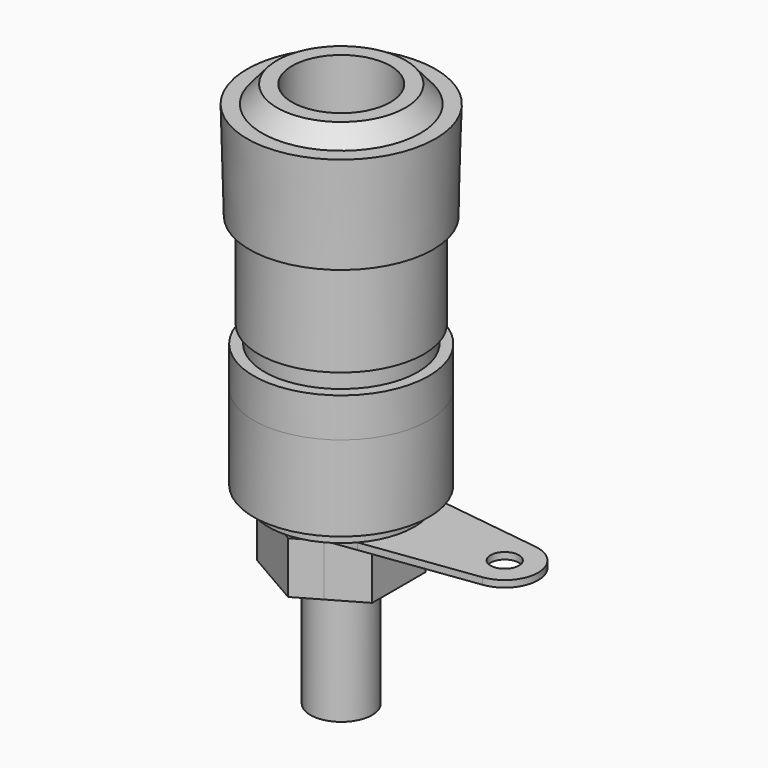
from build123d import *

# Parameters (mm, degrees)
F0_R      = 5.25
F0_R_2    = 3.925
F0_R_3    = 2.4
F1_DEPTH  = 2.35
F2_DEPTH  = 5
F3_DEPTH  = 5.1
F4_R      = 4.6
F4_R_2    = 2.85
F4_R_3    = 2.4
F4_R_4    = 2.35
F4_R_5    = 2
F5_DEPTH  = 1.05
F6_DEPTH  = 9.25
F4_R_6    = 1.85
F7_DEPTH  = 2.5
F8_DEPTH  = 19
F9_DEPTH  = 2.15
F12_R     = 4.375
F12_R_2   = 3.925
F12_R_3   = 2.1
F13_DEPTH = 0.8
F14_R     = 2.1
F14_R_2   = 0.85
F15_DEPTH = 0.4
F16_R     = 2.1
F16_R_2   = 1.7
F17_DEPTH = 3.1


with BuildPart() as f1:
    # F0 (on Top) → F1 (new body)
    with BuildSketch(Plane.XY):
        Circle(F0_R)
        Circle(F0_R_2, mode=Mode.SUBTRACT)
        Circle(F0_R_2)
        Circle(F0_R_3, mode=Mode.SUBTRACT)
    extrude(amount=F1_DEPTH)

    # F0 (on Top) → F2 (join)
    with BuildSketch(Plane.XY):
        Circle(F0_R_2)
        Circle(F0_R_3, mode=Mode.SUBTRACT)
    extrude(amount=-F2_DEPTH)


with BuildPart() as f3:
    # F0 (on Top) → F3 (new body)
    with BuildSketch(Plane.XY):
        Circle(F0_R)
        Circle(F0_R_2, mode=Mode.SUBTRACT)
    extrude(amount=-F3_DEPTH)


with BuildPart() as f5:
    # F4 (on face) → F5 (new body)
    with BuildSketch(Plane.XY.offset(2.35)):
        Circle(F4_R)
        Circle(F4_R_2, mode=Mode.SUBTRACT)
        Circle(F4_R_2)
        Circle(F4_R_3, mode=Mode.SUBTRACT)
        Circle(F4_R_3)
        Circle(F4_R_4, mode=Mode.SUBTRACT)
        Circle(F4_R_4)
        Circle(F4_R_5, mode=Mode.SUBTRACT)
    extrude(amount=F5_DEPTH)

    # F4 (on face) → F6 (join)
    with BuildSketch(Plane.XY.offset(2.35)):
        Circle(F4_R_2)
        Circle(F4_R_3, mode=Mode.SUBTRACT)
        Circle(F4_R_3)
        Circle(F4_R_4, mode=Mode.SUBTRACT)
        Circle(F4_R_4)
        Circle(F4_R_5, mode=Mode.SUBTRACT)
    extrude(amount=F6_DEPTH)

    # F4 (on face) → F7 (join)
    with BuildSketch(Plane.XY.offset(2.35)):
        Circle(F4_R_4)
        Circle(F4_R_5, mode=Mode.SUBTRACT)
        Circle(F4_R_5)
        Circle(F4_R_6, mode=Mode.SUBTRACT)
    extrude(amount=-F7_DEPTH)

    # F4 (on face) → F8 (join)
    with BuildSketch(Plane.XY.offset(2.35)):
        Circle(F4_R_6)
    extrude(amount=-F8_DEPTH)

    # F4 (on face) → F9 (cut)
    with BuildSketch(Plane.XY.offset(2.35)):
        Circle(F4_R_5)
        Circle(F4_R_6, mode=Mode.SUBTRACT)
        Circle(F4_R_6)
    extrude(amount=-F9_DEPTH, mode=Mode.SUBTRACT)


with BuildPart() as f11:
    # F10 (on Front) → F11 (revolve)
    with BuildSketch(Plane.XZ):
        Polygon((3.85, 16.05), (2.95, 16.05), (2.95, 11.55), (2.7, 11.55), (2.7, 6.8), (3.2, 6.8), (3.2, 3.4), (4.95, 3.4), (4.95, 9.1), (5.5, 9.1), (5.65, 15), (4.75, 15), align=None)
    revolve(axis=Axis((0, 0, 12.6171559095), (0, 0, 1)))


with BuildPart() as f13:
    # F12 (on face) → F13 (new body)
    with BuildSketch(Plane(origin=(0, 0, -5.1), x_dir=(1, 0, 0), z_dir=(0, 0, -1))):
        Circle(F12_R)
        Circle(F12_R_2, mode=Mode.SUBTRACT)
        Circle(F12_R_2)
        Circle(F12_R_3, mode=Mode.SUBTRACT)
    extrude(amount=F13_DEPTH)


with BuildPart() as f15:
    # F14 (on face) → F15 (new body)
    with BuildSketch(Plane(origin=(0, 0, -5.9), x_dir=(1, 0, 0), z_dir=(0, 0, -1))):
        with BuildLine():
            Line((0.437755102, -3.2708363564), (3.2847605668, -2.889805014))
            ThreePointArc((3.2847605668, -2.889805014), (4.0933758977, -1.5443117432), (4.375, 0))
            ThreePointArc((4.375, 0), (4.0933758977, 1.5443117432), (3.2847605668, 2.889805014))
            Line((3.2847605668, 2.889805014), (0.437755102, 3.2708363564))
            ThreePointArc((0.437755102, 3.2708363564), (-3.3, 0), (0.437755102, -3.2708363564))
        make_face()
        Circle(F14_R, mode=Mode.SUBTRACT)
        with BuildLine():
            Line((3.2847605668, -2.889805014), (10.0653061224, -1.9823250645))
            ThreePointArc((10.0653061224, -1.9823250645), (11.8, 0), (10.0653061224, 1.9823250645))
            Line((10.0653061224, 1.9823250645), (3.2847605668, 2.889805014))
            ThreePointArc((3.2847605668, 2.889805014), (4.0933758977, 1.5443117432), (4.375, 0))
            ThreePointArc((4.375, 0), (4.0933758977, -1.5443117432), (3.2847605668, -2.889805014))
        make_face()
        with Locations((9.8, 0)):
            Circle(F14_R_2, mode=Mode.SUBTRACT)
    extrude(amount=F15_DEPTH)


with BuildPart() as f17:
    # F16 (on face) → F17 (new body)
    with BuildSketch(Plane(origin=(0, 0, -6.3), x_dir=(1, 0, 0), z_dir=(0, 0, -1))):
        with BuildLine():
            Line((3.45, 1.9918584287), (1.4752466365, 3.1319828147))
            Line((1.4752466365, 3.1319828147), (0.437755102, 3.2708363564))
            ThreePointArc((0.437755102, 3.2708363564), (-3.3, 0), (0.437755102, -3.2708363564))
            Line((0.437755102, -3.2708363564), (1.4752466365, -3.1319828147))
            Line((1.4752466365, -3.1319828147), (3.45, -1.9918584287))
            Line((3.45, -1.9918584287), (3.45, 1.9918584287))
        make_face()
        Circle(F16_R, mode=Mode.SUBTRACT)
        Circle(F16_R)
        Circle(F16_R_2, mode=Mode.SUBTRACT)
        with BuildLine():
            Line((1.4752466365, 3.1319828147), (0, 3.9837168574))
            Line((0, 3.9837168574), (-3.45, 1.9918584287))
            Line((-3.45, 1.9918584287), (-3.45, -1.9918584287))
            Line((-3.45, -1.9918584287), (0, -3.9837168574))
            Line((0, -3.9837168574), (1.4752466365, -3.1319828147))
            Line((1.4752466365, -3.1319828147), (0.437755102, -3.2708363564))
            ThreePointArc((0.437755102, -3.2708363564), (-3.3, 0), (0.437755102, 3.2708363564))
            Line((0.437755102, 3.2708363564), (1.4752466365, 3.1319828147))
        make_face()
    extrude(amount=F17_DEPTH)


solid = Compound([f1.part, f3.part, f5.part, f11.part, f13.part, f15.part, f17.part])
